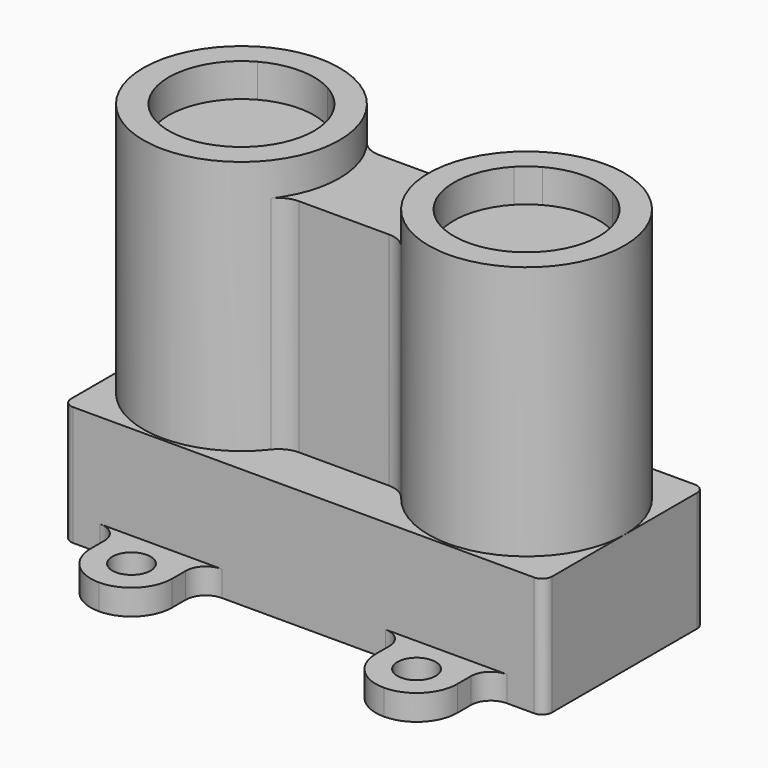
from build123d import *

# Parameters (mm, degrees)
F1_DEPTH    = 2.54
F2_DEPTH    = 11.938
F3_DEPTH    = 34
F4_DEPTH    = 37.338
F5_R        = 1
F6_R        = 2
F7_T1_DEPTH = 25.4067065919


# Not quite as in the source:
# - a fillet or chamfer that OpenCascade refuses, or shapes differently, is made with other operations: its cross-section is extruded or revolved along the edge and cut away or added


with BuildPart() as f1:
    # F0 (on Top) → F1 (new body)
    with BuildSketch(Plane.XY):
        with BuildLine():
            Line((16.129, 13.716), (18.288, 13.716))
            ThreePointArc((18.288, 13.716), (17.0976819587, 16.5896819587), (14.224, 17.78))
            ThreePointArc((14.224, 17.78), (11.3503180413, 16.5896819587), (10.16, 13.716))
            Line((10.16, 13.716), (12.319, 13.716))
            ThreePointArc((12.319, 13.716), (14.224, 15.621), (16.129, 13.716))
        make_face()
        with BuildLine():
            ThreePointArc((-10.16, 13.716), (-11.3503180413, 16.5896819587), (-14.224, 17.78))
            ThreePointArc((-14.224, 17.78), (-17.0976819587, 16.5896819587), (-18.288, 13.716))
            Line((-18.288, 13.716), (-16.129, 13.716))
            ThreePointArc((-16.129, 13.716), (-14.224, 15.621), (-12.319, 13.716))
            Line((-12.319, 13.716), (-10.16, 13.716))
        make_face()
        with BuildLine():
            ThreePointArc((-18.288, -13.716), (-17.0976819587, -16.5896819587), (-14.224, -17.78))
            ThreePointArc((-14.224, -17.78), (-11.3503180413, -16.5896819587), (-10.16, -13.716))
            Line((-10.16, -13.716), (-12.319, -13.716))
            ThreePointArc((-12.319, -13.716), (-14.224, -15.621), (-16.129, -13.716))
            Line((-16.129, -13.716), (-18.288, -13.716))
        make_face()
        with BuildLine():
            ThreePointArc((14.224, -17.78), (17.0976819587, -16.5896819587), (18.288, -13.716))
            Line((18.288, -13.716), (16.129, -13.716))
            ThreePointArc((16.129, -13.716), (14.224, -15.621), (12.319, -13.716))
            Line((12.319, -13.716), (10.16, -13.716))
            ThreePointArc((10.16, -13.716), (11.3503180413, -16.5896819587), (14.224, -17.78))
        make_face()
        with BuildLine():
            ThreePointArc((18.288, -13.716), (17.651692093, -11.5326486963), (15.9420241558, -10.033))
            Line((15.9420241558, -10.033), (12.5059758442, -10.033))
            ThreePointArc((12.5059758442, -10.033), (10.796307907, -11.5326486963), (10.16, -13.716))
            Line((10.16, -13.716), (12.319, -13.716))
            ThreePointArc((12.319, -13.716), (14.224, -11.811), (16.129, -13.716))
            Line((16.129, -13.716), (18.288, -13.716))
        make_face()
        with BuildLine():
            Line((18.288, -13.716), (18.288, -10.033))
            Line((18.288, -10.033), (15.9420241558, -10.033))
            ThreePointArc((15.9420241558, -10.033), (17.651692093, -11.5326486963), (18.288, -13.716))
        make_face()
        with BuildLine():
            ThreePointArc((10.16, -13.716), (10.796307907, -11.5326486963), (12.5059758442, -10.033))
            Line((12.5059758442, -10.033), (10.16, -10.033))
            Line((10.16, -10.033), (10.16, -13.716))
        make_face()
        with BuildLine():
            ThreePointArc((-15.9420241558, -10.033), (-17.651692093, -11.5326486963), (-18.288, -13.716))
            Line((-18.288, -13.716), (-16.129, -13.716))
            ThreePointArc((-16.129, -13.716), (-14.224, -11.811), (-12.319, -13.716))
            Line((-12.319, -13.716), (-10.16, -13.716))
            ThreePointArc((-10.16, -13.716), (-10.796307907, -11.5326486963), (-12.5059758442, -10.033))
            Line((-12.5059758442, -10.033), (-15.9420241558, -10.033))
        make_face()
        with BuildLine():
            Line((-18.288, -10.033), (-18.288, -13.716))
            ThreePointArc((-18.288, -13.716), (-17.651692093, -11.5326486963), (-15.9420241558, -10.033))
            Line((-15.9420241558, -10.033), (-18.288, -10.033))
        make_face()
        with BuildLine():
            ThreePointArc((-12.5059758442, -10.033), (-10.796307907, -11.5326486963), (-10.16, -13.716))
            Line((-10.16, -13.716), (-10.16, -10.033))
            Line((-10.16, -10.033), (-12.5059758442, -10.033))
        make_face()
        with BuildLine():
            Line((12.5059758442, 10.033), (15.9420241558, 10.033))
            ThreePointArc((15.9420241558, 10.033), (17.651692093, 11.5326486963), (18.288, 13.716))
            Line((18.288, 13.716), (16.129, 13.716))
            ThreePointArc((16.129, 13.716), (14.224, 11.811), (12.319, 13.716))
            Line((12.319, 13.716), (10.16, 13.716))
            ThreePointArc((10.16, 13.716), (10.796307907, 11.5326486963), (12.5059758442, 10.033))
        make_face()
        with BuildLine():
            ThreePointArc((-12.5059758442, 10.033), (-10.796307907, 11.5326486963), (-10.16, 13.716))
            Line((-10.16, 13.716), (-12.319, 13.716))
            ThreePointArc((-12.319, 13.716), (-14.224, 11.811), (-16.129, 13.716))
            Line((-16.129, 13.716), (-18.288, 13.716))
            ThreePointArc((-18.288, 13.716), (-17.651692093, 11.5326486963), (-15.9420241558, 10.033))
            Line((-15.9420241558, 10.033), (-12.5059758442, 10.033))
        make_face()
        with BuildLine():
            Line((-8.974, 5), (-5.8199033204, 5))
            ThreePointArc((-5.8199033204, 5), (-7.6929044902, 7.2782987326), (-10.16, 8.8945345578))
            Line((-10.16, 8.8945345578), (-10.16, 6.35))
            Line((-10.16, 6.35), (-10.7254288631, 6.35))
            ThreePointArc((-10.7254288631, 6.35), (-9.7979408912, 5.7421686466), (-8.974, 5))
        make_face()
        with BuildLine():
            Line((-17.7225711369, -6.35), (-10.7254288631, -6.35))
            ThreePointArc((-10.7254288631, -6.35), (-9.7979408912, -5.7421686466), (-8.974, -5))
            Line((-8.974, -5), (-9.5235463232, -5))
            Line((-9.5235463232, -5), (-9.5235463232, 5))
            Line((-9.5235463232, 5), (-8.974, 5))
            ThreePointArc((-8.974, 5), (-9.7979408912, 5.7421686466), (-10.7254288631, 6.35))
            Line((-10.7254288631, 6.35), (-17.7225711369, 6.35))
            ThreePointArc((-17.7225711369, 6.35), (-21.474, 0), (-17.7225711369, -6.35))
        make_face()
        with BuildLine():
            ThreePointArc((-18.288, 8.8945345578), (-22.4511105803, 5.2861604686), (-24.003, 0))
            ThreePointArc((-24.003, 0), (-22.4511105803, -5.2861604686), (-18.288, -8.8945345578))
            Line((-18.288, -8.8945345578), (-18.288, -6.35))
            Line((-18.288, -6.35), (-17.7225711369, -6.35))
            ThreePointArc((-17.7225711369, -6.35), (-21.474, 0), (-17.7225711369, 6.35))
            Line((-17.7225711369, 6.35), (-18.288, 6.35))
            Line((-18.288, 6.35), (-18.288, 8.8945345578))
        make_face()
        with BuildLine():
            ThreePointArc((-15.074346301, 9.7419583333), (-16.7174377184, 9.4557712189), (-18.288, 8.8945345578))
            Line((-18.288, 8.8945345578), (-18.288, 6.35))
            Line((-18.288, 6.35), (-17.7225711369, 6.35))
            ThreePointArc((-17.7225711369, 6.35), (-14.224, 7.25), (-10.7254288631, 6.35))
            Line((-10.7254288631, 6.35), (-10.16, 6.35))
            Line((-10.16, 6.35), (-10.16, 8.8945345578))
            ThreePointArc((-10.16, 8.8945345578), (-11.7305622816, 9.4557712189), (-13.373653699, 9.7419583333))
            ThreePointArc((-13.373653699, 9.7419583333), (-14.224, 9.652), (-15.074346301, 9.7419583333))
        make_face()
        with BuildLine():
            ThreePointArc((-13.373653699, -9.7419583333), (-11.7305622816, -9.4557712189), (-10.16, -8.8945345578))
            Line((-10.16, -8.8945345578), (-10.16, -6.35))
            Line((-10.16, -6.35), (-10.7254288631, -6.35))
            ThreePointArc((-10.7254288631, -6.35), (-14.224, -7.25), (-17.7225711369, -6.35))
            Line((-17.7225711369, -6.35), (-18.288, -6.35))
            Line((-18.288, -6.35), (-18.288, -8.8945345578))
            ThreePointArc((-18.288, -8.8945345578), (-16.7174377184, -9.4557712189), (-15.074346301, -9.7419583333))
            ThreePointArc((-15.074346301, -9.7419583333), (-14.224, -9.652), (-13.373653699, -9.7419583333))
        make_face()
        with BuildLine():
            ThreePointArc((15.074346301, -9.7419583333), (16.7174377184, -9.4557712189), (18.288, -8.8945345578))
            Line((18.288, -8.8945345578), (18.288, -6.35))
            Line((18.288, -6.35), (17.7225711369, -6.35))
            ThreePointArc((17.7225711369, -6.35), (14.224, -7.25), (10.7254288631, -6.35))
            Line((10.7254288631, -6.35), (10.16, -6.35))
            Line((10.16, -6.35), (10.16, -8.8945345578))
            ThreePointArc((10.16, -8.8945345578), (11.7305622816, -9.4557712189), (13.373653699, -9.7419583333))
            ThreePointArc((13.373653699, -9.7419583333), (14.224, -9.652), (15.074346301, -9.7419583333))
        make_face()
        with BuildLine():
            Line((18.288, 6.35), (18.288, 8.8945345578))
            ThreePointArc((18.288, 8.8945345578), (16.7174377184, 9.4557712189), (15.074346301, 9.7419583333))
            ThreePointArc((15.074346301, 9.7419583333), (14.224, 9.652), (13.373653699, 9.7419583333))
            ThreePointArc((13.373653699, 9.7419583333), (11.7305622816, 9.4557712189), (10.16, 8.8945345578))
            Line((10.16, 8.8945345578), (10.16, 6.35))
            Line((10.16, 6.35), (10.7254288631, 6.35))
            ThreePointArc((10.7254288631, 6.35), (14.224, 7.25), (17.7225711369, 6.35))
            Line((17.7225711369, 6.35), (18.288, 6.35))
        make_face()
        with BuildLine():
            Line((10.16, 10.033), (12.5059758442, 10.033))
            ThreePointArc((12.5059758442, 10.033), (10.796307907, 11.5326486963), (10.16, 13.716))
            Line((10.16, 13.716), (10.16, 10.033))
        make_face()
        with BuildLine():
            Line((15.9420241558, 10.033), (18.288, 10.033))
            Line((18.288, 10.033), (18.288, 13.716))
            ThreePointArc((18.288, 13.716), (17.651692093, 11.5326486963), (15.9420241558, 10.033))
        make_face()
        with BuildLine():
            ThreePointArc((13.373653699, 9.7419583333), (14.224, 9.779), (15.074346301, 9.7419583333))
            ThreePointArc((15.074346301, 9.7419583333), (15.5164039669, 9.8629767732), (15.9420241558, 10.033))
            Line((15.9420241558, 10.033), (12.5059758442, 10.033))
            ThreePointArc((12.5059758442, 10.033), (12.9315960331, 9.8629767732), (13.373653699, 9.7419583333))
        make_face()
        with BuildLine():
            Line((12.5059758442, -10.033), (15.9420241558, -10.033))
            ThreePointArc((15.9420241558, -10.033), (15.5164039669, -9.8629767732), (15.074346301, -9.7419583333))
            ThreePointArc((15.074346301, -9.7419583333), (14.224, -9.779), (13.373653699, -9.7419583333))
            ThreePointArc((13.373653699, -9.7419583333), (12.9315960331, -9.8629767732), (12.5059758442, -10.033))
        make_face()
        with BuildLine():
            ThreePointArc((-15.074346301, -9.7419583333), (-15.5164039669, -9.8629767732), (-15.9420241558, -10.033))
            Line((-15.9420241558, -10.033), (-12.5059758442, -10.033))
            ThreePointArc((-12.5059758442, -10.033), (-12.9315960331, -9.8629767732), (-13.373653699, -9.7419583333))
            ThreePointArc((-13.373653699, -9.7419583333), (-14.224, -9.779), (-15.074346301, -9.7419583333))
        make_face()
        with BuildLine():
            ThreePointArc((-13.373653699, 9.7419583333), (-12.9315960331, 9.8629767732), (-12.5059758442, 10.033))
            Line((-12.5059758442, 10.033), (-15.9420241558, 10.033))
            ThreePointArc((-15.9420241558, 10.033), (-15.5164039669, 9.8629767732), (-15.074346301, 9.7419583333))
            ThreePointArc((-15.074346301, 9.7419583333), (-14.224, 9.779), (-13.373653699, 9.7419583333))
        make_face()
        with BuildLine():
            ThreePointArc((-15.9420241558, 10.033), (-17.651692093, 11.5326486963), (-18.288, 13.716))
            Line((-18.288, 13.716), (-18.288, 10.033))
            Line((-18.288, 10.033), (-15.9420241558, 10.033))
        make_face()
        with BuildLine():
            Line((-10.16, 10.033), (-10.16, 13.716))
            ThreePointArc((-10.16, 13.716), (-10.796307907, 11.5326486963), (-12.5059758442, 10.033))
            Line((-12.5059758442, 10.033), (-10.16, 10.033))
        make_face()
        with BuildLine():
            Line((-9.5235463232, -5), (-8.974, -5))
            ThreePointArc((-8.974, -5), (-7.4925439911, -2.6925824036), (-6.974, 0))
            ThreePointArc((-6.974, 0), (-7.4925439911, 2.6925824036), (-8.974, 5))
            Line((-8.974, 5), (-9.5235463232, 5))
            Line((-9.5235463232, 5), (-9.5235463232, -5))
        make_face()
        with BuildLine():
            ThreePointArc((5.8199033204, 5), (7.6929044902, 7.2782987326), (10.16, 8.8945345578))
            Line((10.16, 8.8945345578), (10.16, 10.033))
            Line((10.16, 10.033), (-10.16, 10.033))
            Line((-10.16, 10.033), (-10.16, 8.8945345578))
            ThreePointArc((-10.16, 8.8945345578), (-7.6929044902, 7.2782987326), (-5.8199033204, 5))
            Line((-5.8199033204, 5), (5.8199033204, 5))
        make_face()
        with BuildLine():
            ThreePointArc((8.974, 5), (6.974, 0), (8.974, -5))
            Line((8.974, -5), (9.5235463232, -5))
            Line((9.5235463232, -5), (9.5235463232, 5))
            Line((9.5235463232, 5), (8.974, 5))
        make_face()
        with BuildLine():
            Line((-5.8199033204, -5), (5.8199033204, -5))
            ThreePointArc((5.8199033204, -5), (4.445, 0), (5.8199033204, 5))
            Line((5.8199033204, 5), (-5.8199033204, 5))
            ThreePointArc((-5.8199033204, 5), (-4.7949888528, 2.5927957469), (-4.445, 0))
            ThreePointArc((-4.445, 0), (-4.7949888528, -2.5927957469), (-5.8199033204, -5))
        make_face()
        with BuildLine():
            Line((-10.16, -10.033), (10.16, -10.033))
            Line((10.16, -10.033), (10.16, -8.8945345578))
            ThreePointArc((10.16, -8.8945345578), (7.6929044902, -7.2782987326), (5.8199033204, -5))
            Line((5.8199033204, -5), (-5.8199033204, -5))
            ThreePointArc((-5.8199033204, -5), (-7.6929044902, -7.2782987326), (-10.16, -8.8945345578))
            Line((-10.16, -8.8945345578), (-10.16, -10.033))
        make_face()
        with BuildLine():
            ThreePointArc((18.288, -8.8945345578), (22.4511105803, -5.2861604686), (24.003, 0))
            ThreePointArc((24.003, 0), (22.4511105803, 5.2861604686), (18.288, 8.8945345578))
            Line((18.288, 8.8945345578), (18.288, 6.35))
            Line((18.288, 6.35), (17.7225711369, 6.35))
            ThreePointArc((17.7225711369, 6.35), (20.4660806124, 3.6876726575), (21.474, 0))
            ThreePointArc((21.474, 0), (20.4660806124, -3.6876726575), (17.7225711369, -6.35))
            Line((17.7225711369, -6.35), (18.288, -6.35))
            Line((18.288, -6.35), (18.288, -8.8945345578))
        make_face()
        with BuildLine():
            Line((10.7254288631, -6.35), (17.7225711369, -6.35))
            ThreePointArc((17.7225711369, -6.35), (20.4660806124, -3.6876726575), (21.474, 0))
            ThreePointArc((21.474, 0), (20.4660806124, 3.6876726575), (17.7225711369, 6.35))
            Line((17.7225711369, 6.35), (10.7254288631, 6.35))
            ThreePointArc((10.7254288631, 6.35), (9.7979408912, 5.7421686466), (8.974, 5))
            Line((8.974, 5), (9.5235463232, 5))
            Line((9.5235463232, 5), (9.5235463232, -5))
            Line((9.5235463232, -5), (8.974, -5))
            ThreePointArc((8.974, -5), (9.7979408912, -5.7421686466), (10.7254288631, -6.35))
        make_face()
        with BuildLine():
            ThreePointArc((8.974, 5), (9.7979408912, 5.7421686466), (10.7254288631, 6.35))
            Line((10.7254288631, 6.35), (10.16, 6.35))
            Line((10.16, 6.35), (10.16, 8.8945345578))
            ThreePointArc((10.16, 8.8945345578), (7.6929044902, 7.2782987326), (5.8199033204, 5))
            Line((5.8199033204, 5), (8.974, 5))
        make_face()
        with BuildLine():
            ThreePointArc((-15.074346301, 9.7419583333), (-15.5164039669, 9.8629767732), (-15.9420241558, 10.033))
            Line((-15.9420241558, 10.033), (-18.288, 10.033))
            Line((-18.288, 10.033), (-18.288, 8.8945345578))
            ThreePointArc((-18.288, 8.8945345578), (-16.7174377184, 9.4557712189), (-15.074346301, 9.7419583333))
        make_face()
        with BuildLine():
            ThreePointArc((-15.074346301, 9.7419583333), (-14.224, 9.652), (-13.373653699, 9.7419583333))
            ThreePointArc((-13.373653699, 9.7419583333), (-14.224, 9.779), (-15.074346301, 9.7419583333))
        make_face()
        with BuildLine():
            Line((-10.16, 8.8945345578), (-10.16, 10.033))
            Line((-10.16, 10.033), (-12.5059758442, 10.033))
            ThreePointArc((-12.5059758442, 10.033), (-12.9315960331, 9.8629767732), (-13.373653699, 9.7419583333))
            ThreePointArc((-13.373653699, 9.7419583333), (-11.7305622816, 9.4557712189), (-10.16, 8.8945345578))
        make_face()
        with BuildLine():
            Line((-18.288, -10.033), (-15.9420241558, -10.033))
            ThreePointArc((-15.9420241558, -10.033), (-15.5164039669, -9.8629767732), (-15.074346301, -9.7419583333))
            ThreePointArc((-15.074346301, -9.7419583333), (-16.7174377184, -9.4557712189), (-18.288, -8.8945345578))
            Line((-18.288, -8.8945345578), (-18.288, -10.033))
        make_face()
        with BuildLine():
            ThreePointArc((-13.373653699, -9.7419583333), (-14.224, -9.652), (-15.074346301, -9.7419583333))
            ThreePointArc((-15.074346301, -9.7419583333), (-14.224, -9.779), (-13.373653699, -9.7419583333))
        make_face()
        with BuildLine():
            Line((-12.5059758442, -10.033), (-10.16, -10.033))
            Line((-10.16, -10.033), (-10.16, -8.8945345578))
            ThreePointArc((-10.16, -8.8945345578), (-11.7305622816, -9.4557712189), (-13.373653699, -9.7419583333))
            ThreePointArc((-13.373653699, -9.7419583333), (-12.9315960331, -9.8629767732), (-12.5059758442, -10.033))
        make_face()
        with BuildLine():
            Line((15.9420241558, -10.033), (18.288, -10.033))
            Line((18.288, -10.033), (18.288, -8.8945345578))
            ThreePointArc((18.288, -8.8945345578), (16.7174377184, -9.4557712189), (15.074346301, -9.7419583333))
            ThreePointArc((15.074346301, -9.7419583333), (15.5164039669, -9.8629767732), (15.9420241558, -10.033))
        make_face()
        with BuildLine():
            Line((10.16, -10.033), (12.5059758442, -10.033))
            ThreePointArc((12.5059758442, -10.033), (12.9315960331, -9.8629767732), (13.373653699, -9.7419583333))
            ThreePointArc((13.373653699, -9.7419583333), (11.7305622816, -9.4557712189), (10.16, -8.8945345578))
            Line((10.16, -8.8945345578), (10.16, -10.033))
        make_face()
        with BuildLine():
            ThreePointArc((13.373653699, -9.7419583333), (14.224, -9.779), (15.074346301, -9.7419583333))
            ThreePointArc((15.074346301, -9.7419583333), (14.224, -9.652), (13.373653699, -9.7419583333))
        make_face()
        with BuildLine():
            ThreePointArc((13.373653699, 9.7419583333), (14.224, 9.652), (15.074346301, 9.7419583333))
            ThreePointArc((15.074346301, 9.7419583333), (14.224, 9.779), (13.373653699, 9.7419583333))
        make_face()
        with BuildLine():
            ThreePointArc((10.16, 8.8945345578), (11.7305622816, 9.4557712189), (13.373653699, 9.7419583333))
            ThreePointArc((13.373653699, 9.7419583333), (12.9315960331, 9.8629767732), (12.5059758442, 10.033))
            Line((12.5059758442, 10.033), (10.16, 10.033))
            Line((10.16, 10.033), (10.16, 8.8945345578))
        make_face()
        with BuildLine():
            ThreePointArc((15.074346301, 9.7419583333), (16.7174377184, 9.4557712189), (18.288, 8.8945345578))
            Line((18.288, 8.8945345578), (18.288, 10.033))
            Line((18.288, 10.033), (15.9420241558, 10.033))
            ThreePointArc((15.9420241558, 10.033), (15.5164039669, 9.8629767732), (15.074346301, 9.7419583333))
        make_face()
        with BuildLine():
            Line((18.288, -10.033), (24.003, -10.033))
            Line((24.003, -10.033), (24.003, 0))
            ThreePointArc((24.003, 0), (22.4511105803, -5.2861604686), (18.288, -8.8945345578))
            Line((18.288, -8.8945345578), (18.288, -10.033))
        make_face()
        with BuildLine():
            ThreePointArc((18.288, 8.8945345578), (22.4511105803, 5.2861604686), (24.003, 0))
            Line((24.003, 0), (24.003, 10.033))
            Line((24.003, 10.033), (18.288, 10.033))
            Line((18.288, 10.033), (18.288, 8.8945345578))
        make_face()
        with BuildLine():
            Line((-24.003, 0), (-24.003, -10.033))
            Line((-24.003, -10.033), (-18.288, -10.033))
            Line((-18.288, -10.033), (-18.288, -8.8945345578))
            ThreePointArc((-18.288, -8.8945345578), (-22.4511105803, -5.2861604686), (-24.003, 0))
        make_face()
        with BuildLine():
            Line((-24.003, 10.033), (-24.003, 0))
            ThreePointArc((-24.003, 0), (-22.4511105803, 5.2861604686), (-18.288, 8.8945345578))
            Line((-18.288, 8.8945345578), (-18.288, 10.033))
            Line((-18.288, 10.033), (-24.003, 10.033))
        make_face()
        with BuildLine():
            Line((-8.974, -5), (-5.8199033204, -5))
            ThreePointArc((-5.8199033204, -5), (-4.7949888528, -2.5927957469), (-4.445, 0))
            ThreePointArc((-4.445, 0), (-4.7949888528, 2.5927957469), (-5.8199033204, 5))
            Line((-5.8199033204, 5), (-8.974, 5))
            ThreePointArc((-8.974, 5), (-7.4925439911, 2.6925824036), (-6.974, 0))
            ThreePointArc((-6.974, 0), (-7.4925439911, -2.6925824036), (-8.974, -5))
        make_face()
        with BuildLine():
            ThreePointArc((-17.7225711369, -6.35), (-14.224, -7.25), (-10.7254288631, -6.35))
            Line((-10.7254288631, -6.35), (-17.7225711369, -6.35))
        make_face()
        with BuildLine():
            Line((-17.7225711369, 6.35), (-10.7254288631, 6.35))
            ThreePointArc((-10.7254288631, 6.35), (-14.224, 7.25), (-17.7225711369, 6.35))
        make_face()
        with BuildLine():
            Line((-10.16, -6.35), (-10.16, -8.8945345578))
            ThreePointArc((-10.16, -8.8945345578), (-7.6929044902, -7.2782987326), (-5.8199033204, -5))
            Line((-5.8199033204, -5), (-8.974, -5))
            ThreePointArc((-8.974, -5), (-9.7979408912, -5.7421686466), (-10.7254288631, -6.35))
            Line((-10.7254288631, -6.35), (-10.16, -6.35))
        make_face()
        with BuildLine():
            ThreePointArc((5.8199033204, 5), (4.445, 0), (5.8199033204, -5))
            Line((5.8199033204, -5), (8.974, -5))
            ThreePointArc((8.974, -5), (6.974, 0), (8.974, 5))
            Line((8.974, 5), (5.8199033204, 5))
        make_face()
        with BuildLine():
            ThreePointArc((5.8199033204, -5), (7.6929044902, -7.2782987326), (10.16, -8.8945345578))
            Line((10.16, -8.8945345578), (10.16, -6.35))
            Line((10.16, -6.35), (10.7254288631, -6.35))
            ThreePointArc((10.7254288631, -6.35), (9.7979408912, -5.7421686466), (8.974, -5))
            Line((8.974, -5), (5.8199033204, -5))
        make_face()
        with BuildLine():
            ThreePointArc((10.7254288631, -6.35), (14.224, -7.25), (17.7225711369, -6.35))
            Line((17.7225711369, -6.35), (10.7254288631, -6.35))
        make_face()
        with BuildLine():
            Line((10.7254288631, 6.35), (17.7225711369, 6.35))
            ThreePointArc((17.7225711369, 6.35), (14.224, 7.25), (10.7254288631, 6.35))
        make_face()
    extrude(amount=F1_DEPTH)

    # F0 (on Top) → F2 (join)
    with BuildSketch(Plane.XY):
        with BuildLine():
            Line((-8.974, 5), (-5.8199033204, 5))
            ThreePointArc((-5.8199033204, 5), (-7.6929044902, 7.2782987326), (-10.16, 8.8945345578))
            Line((-10.16, 8.8945345578), (-10.16, 6.35))
            Line((-10.16, 6.35), (-10.7254288631, 6.35))
            ThreePointArc((-10.7254288631, 6.35), (-9.7979408912, 5.7421686466), (-8.974, 5))
        make_face()
        with BuildLine():
            Line((-17.7225711369, -6.35), (-10.7254288631, -6.35))
            ThreePointArc((-10.7254288631, -6.35), (-9.7979408912, -5.7421686466), (-8.974, -5))
            Line((-8.974, -5), (-9.5235463232, -5))
            Line((-9.5235463232, -5), (-9.5235463232, 5))
            Line((-9.5235463232, 5), (-8.974, 5))
            ThreePointArc((-8.974, 5), (-9.7979408912, 5.7421686466), (-10.7254288631, 6.35))
            Line((-10.7254288631, 6.35), (-17.7225711369, 6.35))
            ThreePointArc((-17.7225711369, 6.35), (-21.474, 0), (-17.7225711369, -6.35))
        make_face()
        with BuildLine():
            ThreePointArc((-18.288, 8.8945345578), (-22.4511105803, 5.2861604686), (-24.003, 0))
            ThreePointArc((-24.003, 0), (-22.4511105803, -5.2861604686), (-18.288, -8.8945345578))
            Line((-18.288, -8.8945345578), (-18.288, -6.35))
            Line((-18.288, -6.35), (-17.7225711369, -6.35))
            ThreePointArc((-17.7225711369, -6.35), (-21.474, 0), (-17.7225711369, 6.35))
            Line((-17.7225711369, 6.35), (-18.288, 6.35))
            Line((-18.288, 6.35), (-18.288, 8.8945345578))
        make_face()
        with BuildLine():
            ThreePointArc((-13.373653699, -9.7419583333), (-11.7305622816, -9.4557712189), (-10.16, -8.8945345578))
            Line((-10.16, -8.8945345578), (-10.16, -6.35))
            Line((-10.16, -6.35), (-10.7254288631, -6.35))
            ThreePointArc((-10.7254288631, -6.35), (-14.224, -7.25), (-17.7225711369, -6.35))
            Line((-17.7225711369, -6.35), (-18.288, -6.35))
            Line((-18.288, -6.35), (-18.288, -8.8945345578))
            ThreePointArc((-18.288, -8.8945345578), (-16.7174377184, -9.4557712189), (-15.074346301, -9.7419583333))
            ThreePointArc((-15.074346301, -9.7419583333), (-14.224, -9.652), (-13.373653699, -9.7419583333))
        make_face()
        with BuildLine():
            ThreePointArc((15.074346301, -9.7419583333), (16.7174377184, -9.4557712189), (18.288, -8.8945345578))
            Line((18.288, -8.8945345578), (18.288, -6.35))
            Line((18.288, -6.35), (17.7225711369, -6.35))
            ThreePointArc((17.7225711369, -6.35), (14.224, -7.25), (10.7254288631, -6.35))
            Line((10.7254288631, -6.35), (10.16, -6.35))
            Line((10.16, -6.35), (10.16, -8.8945345578))
            ThreePointArc((10.16, -8.8945345578), (11.7305622816, -9.4557712189), (13.373653699, -9.7419583333))
            ThreePointArc((13.373653699, -9.7419583333), (14.224, -9.652), (15.074346301, -9.7419583333))
        make_face()
        with BuildLine():
            Line((18.288, 6.35), (18.288, 8.8945345578))
            ThreePointArc((18.288, 8.8945345578), (16.7174377184, 9.4557712189), (15.074346301, 9.7419583333))
            ThreePointArc((15.074346301, 9.7419583333), (14.224, 9.652), (13.373653699, 9.7419583333))
            ThreePointArc((13.373653699, 9.7419583333), (11.7305622816, 9.4557712189), (10.16, 8.8945345578))
            Line((10.16, 8.8945345578), (10.16, 6.35))
            Line((10.16, 6.35), (10.7254288631, 6.35))
            ThreePointArc((10.7254288631, 6.35), (14.224, 7.25), (17.7225711369, 6.35))
            Line((17.7225711369, 6.35), (18.288, 6.35))
        make_face()
        with BuildLine():
            Line((12.5059758442, -10.033), (15.9420241558, -10.033))
            ThreePointArc((15.9420241558, -10.033), (15.5164039669, -9.8629767732), (15.074346301, -9.7419583333))
            ThreePointArc((15.074346301, -9.7419583333), (14.224, -9.779), (13.373653699, -9.7419583333))
            ThreePointArc((13.373653699, -9.7419583333), (12.9315960331, -9.8629767732), (12.5059758442, -10.033))
        make_face()
        with BuildLine():
            ThreePointArc((13.373653699, 9.7419583333), (14.224, 9.779), (15.074346301, 9.7419583333))
            ThreePointArc((15.074346301, 9.7419583333), (15.5164039669, 9.8629767732), (15.9420241558, 10.033))
            Line((15.9420241558, 10.033), (12.5059758442, 10.033))
            ThreePointArc((12.5059758442, 10.033), (12.9315960331, 9.8629767732), (13.373653699, 9.7419583333))
        make_face()
        with BuildLine():
            ThreePointArc((-15.074346301, -9.7419583333), (-15.5164039669, -9.8629767732), (-15.9420241558, -10.033))
            Line((-15.9420241558, -10.033), (-12.5059758442, -10.033))
            ThreePointArc((-12.5059758442, -10.033), (-12.9315960331, -9.8629767732), (-13.373653699, -9.7419583333))
            ThreePointArc((-13.373653699, -9.7419583333), (-14.224, -9.779), (-15.074346301, -9.7419583333))
        make_face()
        with BuildLine():
            ThreePointArc((-13.373653699, 9.7419583333), (-12.9315960331, 9.8629767732), (-12.5059758442, 10.033))
            Line((-12.5059758442, 10.033), (-15.9420241558, 10.033))
            ThreePointArc((-15.9420241558, 10.033), (-15.5164039669, 9.8629767732), (-15.074346301, 9.7419583333))
            ThreePointArc((-15.074346301, 9.7419583333), (-14.224, 9.779), (-13.373653699, 9.7419583333))
        make_face()
        with BuildLine():
            Line((-24.003, 10.033), (-24.003, 0))
            ThreePointArc((-24.003, 0), (-22.4511105803, 5.2861604686), (-18.288, 8.8945345578))
            Line((-18.288, 8.8945345578), (-18.288, 10.033))
            Line((-18.288, 10.033), (-24.003, 10.033))
        make_face()
        with BuildLine():
            Line((-24.003, 0), (-24.003, -10.033))
            Line((-24.003, -10.033), (-18.288, -10.033))
            Line((-18.288, -10.033), (-18.288, -8.8945345578))
            ThreePointArc((-18.288, -8.8945345578), (-22.4511105803, -5.2861604686), (-24.003, 0))
        make_face()
        with BuildLine():
            Line((-10.16, -10.033), (10.16, -10.033))
            Line((10.16, -10.033), (10.16, -8.8945345578))
            ThreePointArc((10.16, -8.8945345578), (7.6929044902, -7.2782987326), (5.8199033204, -5))
            Line((5.8199033204, -5), (-5.8199033204, -5))
            ThreePointArc((-5.8199033204, -5), (-7.6929044902, -7.2782987326), (-10.16, -8.8945345578))
            Line((-10.16, -8.8945345578), (-10.16, -10.033))
        make_face()
        with BuildLine():
            Line((-9.5235463232, -5), (-8.974, -5))
            ThreePointArc((-8.974, -5), (-7.4925439911, -2.6925824036), (-6.974, 0))
            ThreePointArc((-6.974, 0), (-7.4925439911, 2.6925824036), (-8.974, 5))
            Line((-8.974, 5), (-9.5235463232, 5))
            Line((-9.5235463232, 5), (-9.5235463232, -5))
        make_face()
        with BuildLine():
            Line((-5.8199033204, -5), (5.8199033204, -5))
            ThreePointArc((5.8199033204, -5), (4.445, 0), (5.8199033204, 5))
            Line((5.8199033204, 5), (-5.8199033204, 5))
            ThreePointArc((-5.8199033204, 5), (-4.7949888528, 2.5927957469), (-4.445, 0))
            ThreePointArc((-4.445, 0), (-4.7949888528, -2.5927957469), (-5.8199033204, -5))
        make_face()
        with BuildLine():
            ThreePointArc((8.974, 5), (6.974, 0), (8.974, -5))
            Line((8.974, -5), (9.5235463232, -5))
            Line((9.5235463232, -5), (9.5235463232, 5))
            Line((9.5235463232, 5), (8.974, 5))
        make_face()
        with BuildLine():
            ThreePointArc((18.288, -8.8945345578), (22.4511105803, -5.2861604686), (24.003, 0))
            ThreePointArc((24.003, 0), (22.4511105803, 5.2861604686), (18.288, 8.8945345578))
            Line((18.288, 8.8945345578), (18.288, 6.35))
            Line((18.288, 6.35), (17.7225711369, 6.35))
            ThreePointArc((17.7225711369, 6.35), (20.4660806124, 3.6876726575), (21.474, 0))
            ThreePointArc((21.474, 0), (20.4660806124, -3.6876726575), (17.7225711369, -6.35))
            Line((17.7225711369, -6.35), (18.288, -6.35))
            Line((18.288, -6.35), (18.288, -8.8945345578))
        make_face()
        with BuildLine():
            Line((10.7254288631, -6.35), (17.7225711369, -6.35))
            ThreePointArc((17.7225711369, -6.35), (20.4660806124, -3.6876726575), (21.474, 0))
            ThreePointArc((21.474, 0), (20.4660806124, 3.6876726575), (17.7225711369, 6.35))
            Line((17.7225711369, 6.35), (10.7254288631, 6.35))
            ThreePointArc((10.7254288631, 6.35), (9.7979408912, 5.7421686466), (8.974, 5))
            Line((8.974, 5), (9.5235463232, 5))
            Line((9.5235463232, 5), (9.5235463232, -5))
            Line((9.5235463232, -5), (8.974, -5))
            ThreePointArc((8.974, -5), (9.7979408912, -5.7421686466), (10.7254288631, -6.35))
        make_face()
        with BuildLine():
            ThreePointArc((8.974, 5), (9.7979408912, 5.7421686466), (10.7254288631, 6.35))
            Line((10.7254288631, 6.35), (10.16, 6.35))
            Line((10.16, 6.35), (10.16, 8.8945345578))
            ThreePointArc((10.16, 8.8945345578), (7.6929044902, 7.2782987326), (5.8199033204, 5))
            Line((5.8199033204, 5), (8.974, 5))
        make_face()
        with BuildLine():
            ThreePointArc((18.288, 8.8945345578), (22.4511105803, 5.2861604686), (24.003, 0))
            Line((24.003, 0), (24.003, 10.033))
            Line((24.003, 10.033), (18.288, 10.033))
            Line((18.288, 10.033), (18.288, 8.8945345578))
        make_face()
        with BuildLine():
            Line((18.288, -10.033), (24.003, -10.033))
            Line((24.003, -10.033), (24.003, 0))
            ThreePointArc((24.003, 0), (22.4511105803, -5.2861604686), (18.288, -8.8945345578))
            Line((18.288, -8.8945345578), (18.288, -10.033))
        make_face()
        with BuildLine():
            ThreePointArc((5.8199033204, 5), (7.6929044902, 7.2782987326), (10.16, 8.8945345578))
            Line((10.16, 8.8945345578), (10.16, 10.033))
            Line((10.16, 10.033), (-10.16, 10.033))
            Line((-10.16, 10.033), (-10.16, 8.8945345578))
            ThreePointArc((-10.16, 8.8945345578), (-7.6929044902, 7.2782987326), (-5.8199033204, 5))
            Line((-5.8199033204, 5), (5.8199033204, 5))
        make_face()
        with BuildLine():
            Line((-12.5059758442, -10.033), (-10.16, -10.033))
            Line((-10.16, -10.033), (-10.16, -8.8945345578))
            ThreePointArc((-10.16, -8.8945345578), (-11.7305622816, -9.4557712189), (-13.373653699, -9.7419583333))
            ThreePointArc((-13.373653699, -9.7419583333), (-12.9315960331, -9.8629767732), (-12.5059758442, -10.033))
        make_face()
        with BuildLine():
            Line((-18.288, -10.033), (-15.9420241558, -10.033))
            ThreePointArc((-15.9420241558, -10.033), (-15.5164039669, -9.8629767732), (-15.074346301, -9.7419583333))
            ThreePointArc((-15.074346301, -9.7419583333), (-16.7174377184, -9.4557712189), (-18.288, -8.8945345578))
            Line((-18.288, -8.8945345578), (-18.288, -10.033))
        make_face()
        with BuildLine():
            ThreePointArc((-13.373653699, -9.7419583333), (-14.224, -9.652), (-15.074346301, -9.7419583333))
            ThreePointArc((-15.074346301, -9.7419583333), (-14.224, -9.779), (-13.373653699, -9.7419583333))
        make_face()
        with BuildLine():
            Line((-10.16, 8.8945345578), (-10.16, 10.033))
            Line((-10.16, 10.033), (-12.5059758442, 10.033))
            ThreePointArc((-12.5059758442, 10.033), (-12.9315960331, 9.8629767732), (-13.373653699, 9.7419583333))
            ThreePointArc((-13.373653699, 9.7419583333), (-11.7305622816, 9.4557712189), (-10.16, 8.8945345578))
        make_face()
        with BuildLine():
            ThreePointArc((-15.074346301, 9.7419583333), (-15.5164039669, 9.8629767732), (-15.9420241558, 10.033))
            Line((-15.9420241558, 10.033), (-18.288, 10.033))
            Line((-18.288, 10.033), (-18.288, 8.8945345578))
            ThreePointArc((-18.288, 8.8945345578), (-16.7174377184, 9.4557712189), (-15.074346301, 9.7419583333))
        make_face()
        with BuildLine():
            ThreePointArc((-15.074346301, 9.7419583333), (-14.224, 9.652), (-13.373653699, 9.7419583333))
            ThreePointArc((-13.373653699, 9.7419583333), (-14.224, 9.779), (-15.074346301, 9.7419583333))
        make_face()
        with BuildLine():
            ThreePointArc((-15.074346301, 9.7419583333), (-16.7174377184, 9.4557712189), (-18.288, 8.8945345578))
            Line((-18.288, 8.8945345578), (-18.288, 6.35))
            Line((-18.288, 6.35), (-17.7225711369, 6.35))
            ThreePointArc((-17.7225711369, 6.35), (-14.224, 7.25), (-10.7254288631, 6.35))
            Line((-10.7254288631, 6.35), (-10.16, 6.35))
            Line((-10.16, 6.35), (-10.16, 8.8945345578))
            ThreePointArc((-10.16, 8.8945345578), (-11.7305622816, 9.4557712189), (-13.373653699, 9.7419583333))
            ThreePointArc((-13.373653699, 9.7419583333), (-14.224, 9.652), (-15.074346301, 9.7419583333))
        make_face()
        with BuildLine():
            Line((15.9420241558, -10.033), (18.288, -10.033))
            Line((18.288, -10.033), (18.288, -8.8945345578))
            ThreePointArc((18.288, -8.8945345578), (16.7174377184, -9.4557712189), (15.074346301, -9.7419583333))
            ThreePointArc((15.074346301, -9.7419583333), (15.5164039669, -9.8629767732), (15.9420241558, -10.033))
        make_face()
        with BuildLine():
            Line((10.16, -10.033), (12.5059758442, -10.033))
            ThreePointArc((12.5059758442, -10.033), (12.9315960331, -9.8629767732), (13.373653699, -9.7419583333))
            ThreePointArc((13.373653699, -9.7419583333), (11.7305622816, -9.4557712189), (10.16, -8.8945345578))
            Line((10.16, -8.8945345578), (10.16, -10.033))
        make_face()
        with BuildLine():
            ThreePointArc((13.373653699, -9.7419583333), (14.224, -9.779), (15.074346301, -9.7419583333))
            ThreePointArc((15.074346301, -9.7419583333), (14.224, -9.652), (13.373653699, -9.7419583333))
        make_face()
        with BuildLine():
            ThreePointArc((15.074346301, 9.7419583333), (16.7174377184, 9.4557712189), (18.288, 8.8945345578))
            Line((18.288, 8.8945345578), (18.288, 10.033))
            Line((18.288, 10.033), (15.9420241558, 10.033))
            ThreePointArc((15.9420241558, 10.033), (15.5164039669, 9.8629767732), (15.074346301, 9.7419583333))
        make_face()
        with BuildLine():
            ThreePointArc((10.16, 8.8945345578), (11.7305622816, 9.4557712189), (13.373653699, 9.7419583333))
            ThreePointArc((13.373653699, 9.7419583333), (12.9315960331, 9.8629767732), (12.5059758442, 10.033))
            Line((12.5059758442, 10.033), (10.16, 10.033))
            Line((10.16, 10.033), (10.16, 8.8945345578))
        make_face()
        with BuildLine():
            ThreePointArc((13.373653699, 9.7419583333), (14.224, 9.652), (15.074346301, 9.7419583333))
            ThreePointArc((15.074346301, 9.7419583333), (14.224, 9.779), (13.373653699, 9.7419583333))
        make_face()
        with BuildLine():
            Line((-17.7225711369, 6.35), (-10.7254288631, 6.35))
            ThreePointArc((-10.7254288631, 6.35), (-14.224, 7.25), (-17.7225711369, 6.35))
        make_face()
        with BuildLine():
            ThreePointArc((-17.7225711369, -6.35), (-14.224, -7.25), (-10.7254288631, -6.35))
            Line((-10.7254288631, -6.35), (-17.7225711369, -6.35))
        make_face()
        with BuildLine():
            Line((-8.974, -5), (-5.8199033204, -5))
            ThreePointArc((-5.8199033204, -5), (-4.7949888528, -2.5927957469), (-4.445, 0))
            ThreePointArc((-4.445, 0), (-4.7949888528, 2.5927957469), (-5.8199033204, 5))
            Line((-5.8199033204, 5), (-8.974, 5))
            ThreePointArc((-8.974, 5), (-7.4925439911, 2.6925824036), (-6.974, 0))
            ThreePointArc((-6.974, 0), (-7.4925439911, -2.6925824036), (-8.974, -5))
        make_face()
        with BuildLine():
            ThreePointArc((5.8199033204, 5), (4.445, 0), (5.8199033204, -5))
            Line((5.8199033204, -5), (8.974, -5))
            ThreePointArc((8.974, -5), (6.974, 0), (8.974, 5))
            Line((8.974, 5), (5.8199033204, 5))
        make_face()
        with BuildLine():
            Line((10.7254288631, 6.35), (17.7225711369, 6.35))
            ThreePointArc((17.7225711369, 6.35), (14.224, 7.25), (10.7254288631, 6.35))
        make_face()
        with BuildLine():
            ThreePointArc((10.7254288631, -6.35), (14.224, -7.25), (17.7225711369, -6.35))
            Line((17.7225711369, -6.35), (10.7254288631, -6.35))
        make_face()
        with BuildLine():
            ThreePointArc((5.8199033204, -5), (7.6929044902, -7.2782987326), (10.16, -8.8945345578))
            Line((10.16, -8.8945345578), (10.16, -6.35))
            Line((10.16, -6.35), (10.7254288631, -6.35))
            ThreePointArc((10.7254288631, -6.35), (9.7979408912, -5.7421686466), (8.974, -5))
            Line((8.974, -5), (5.8199033204, -5))
        make_face()
        with BuildLine():
            Line((-10.16, -6.35), (-10.16, -8.8945345578))
            ThreePointArc((-10.16, -8.8945345578), (-7.6929044902, -7.2782987326), (-5.8199033204, -5))
            Line((-5.8199033204, -5), (-8.974, -5))
            ThreePointArc((-8.974, -5), (-9.7979408912, -5.7421686466), (-10.7254288631, -6.35))
            Line((-10.7254288631, -6.35), (-10.16, -6.35))
        make_face()
    extrude(amount=F2_DEPTH)

    # F0 (on Top) → F3 (join)
    with BuildSketch(Plane.XY):
        with BuildLine():
            ThreePointArc((-18.288, 8.8945345578), (-22.4511105803, 5.2861604686), (-24.003, 0))
            ThreePointArc((-24.003, 0), (-22.4511105803, -5.2861604686), (-18.288, -8.8945345578))
            Line((-18.288, -8.8945345578), (-18.288, -6.35))
            Line((-18.288, -6.35), (-17.7225711369, -6.35))
            ThreePointArc((-17.7225711369, -6.35), (-21.474, 0), (-17.7225711369, 6.35))
            Line((-17.7225711369, 6.35), (-18.288, 6.35))
            Line((-18.288, 6.35), (-18.288, 8.8945345578))
        make_face()
        with BuildLine():
            ThreePointArc((-15.074346301, 9.7419583333), (-16.7174377184, 9.4557712189), (-18.288, 8.8945345578))
            Line((-18.288, 8.8945345578), (-18.288, 6.35))
            Line((-18.288, 6.35), (-17.7225711369, 6.35))
            ThreePointArc((-17.7225711369, 6.35), (-14.224, 7.25), (-10.7254288631, 6.35))
            Line((-10.7254288631, 6.35), (-10.16, 6.35))
            Line((-10.16, 6.35), (-10.16, 8.8945345578))
            ThreePointArc((-10.16, 8.8945345578), (-11.7305622816, 9.4557712189), (-13.373653699, 9.7419583333))
            ThreePointArc((-13.373653699, 9.7419583333), (-14.224, 9.652), (-15.074346301, 9.7419583333))
        make_face()
        with BuildLine():
            Line((-8.974, 5), (-5.8199033204, 5))
            ThreePointArc((-5.8199033204, 5), (-7.6929044902, 7.2782987326), (-10.16, 8.8945345578))
            Line((-10.16, 8.8945345578), (-10.16, 6.35))
            Line((-10.16, 6.35), (-10.7254288631, 6.35))
            ThreePointArc((-10.7254288631, 6.35), (-9.7979408912, 5.7421686466), (-8.974, 5))
        make_face()
        with BuildLine():
            Line((-8.974, -5), (-5.8199033204, -5))
            ThreePointArc((-5.8199033204, -5), (-4.7949888528, -2.5927957469), (-4.445, 0))
            ThreePointArc((-4.445, 0), (-4.7949888528, 2.5927957469), (-5.8199033204, 5))
            Line((-5.8199033204, 5), (-8.974, 5))
            ThreePointArc((-8.974, 5), (-7.4925439911, 2.6925824036), (-6.974, 0))
            ThreePointArc((-6.974, 0), (-7.4925439911, -2.6925824036), (-8.974, -5))
        make_face()
        with BuildLine():
            Line((-5.8199033204, -5), (5.8199033204, -5))
            ThreePointArc((5.8199033204, -5), (4.445, 0), (5.8199033204, 5))
            Line((5.8199033204, 5), (-5.8199033204, 5))
            ThreePointArc((-5.8199033204, 5), (-4.7949888528, 2.5927957469), (-4.445, 0))
            ThreePointArc((-4.445, 0), (-4.7949888528, -2.5927957469), (-5.8199033204, -5))
        make_face()
        with BuildLine():
            Line((-10.16, -6.35), (-10.16, -8.8945345578))
            ThreePointArc((-10.16, -8.8945345578), (-7.6929044902, -7.2782987326), (-5.8199033204, -5))
            Line((-5.8199033204, -5), (-8.974, -5))
            ThreePointArc((-8.974, -5), (-9.7979408912, -5.7421686466), (-10.7254288631, -6.35))
            Line((-10.7254288631, -6.35), (-10.16, -6.35))
        make_face()
        with BuildLine():
            ThreePointArc((-13.373653699, -9.7419583333), (-11.7305622816, -9.4557712189), (-10.16, -8.8945345578))
            Line((-10.16, -8.8945345578), (-10.16, -6.35))
            Line((-10.16, -6.35), (-10.7254288631, -6.35))
            ThreePointArc((-10.7254288631, -6.35), (-14.224, -7.25), (-17.7225711369, -6.35))
            Line((-17.7225711369, -6.35), (-18.288, -6.35))
            Line((-18.288, -6.35), (-18.288, -8.8945345578))
            ThreePointArc((-18.288, -8.8945345578), (-16.7174377184, -9.4557712189), (-15.074346301, -9.7419583333))
            ThreePointArc((-15.074346301, -9.7419583333), (-14.224, -9.652), (-13.373653699, -9.7419583333))
        make_face()
        with BuildLine():
            ThreePointArc((5.8199033204, 5), (4.445, 0), (5.8199033204, -5))
            Line((5.8199033204, -5), (8.974, -5))
            ThreePointArc((8.974, -5), (6.974, 0), (8.974, 5))
            Line((8.974, 5), (5.8199033204, 5))
        make_face()
        with BuildLine():
            ThreePointArc((8.974, 5), (9.7979408912, 5.7421686466), (10.7254288631, 6.35))
            Line((10.7254288631, 6.35), (10.16, 6.35))
            Line((10.16, 6.35), (10.16, 8.8945345578))
            ThreePointArc((10.16, 8.8945345578), (7.6929044902, 7.2782987326), (5.8199033204, 5))
            Line((5.8199033204, 5), (8.974, 5))
        make_face()
        with BuildLine():
            ThreePointArc((18.288, -8.8945345578), (22.4511105803, -5.2861604686), (24.003, 0))
            ThreePointArc((24.003, 0), (22.4511105803, 5.2861604686), (18.288, 8.8945345578))
            Line((18.288, 8.8945345578), (18.288, 6.35))
            Line((18.288, 6.35), (17.7225711369, 6.35))
            ThreePointArc((17.7225711369, 6.35), (20.4660806124, 3.6876726575), (21.474, 0))
            ThreePointArc((21.474, 0), (20.4660806124, -3.6876726575), (17.7225711369, -6.35))
            Line((17.7225711369, -6.35), (18.288, -6.35))
            Line((18.288, -6.35), (18.288, -8.8945345578))
        make_face()
        with BuildLine():
            ThreePointArc((15.074346301, -9.7419583333), (16.7174377184, -9.4557712189), (18.288, -8.8945345578))
            Line((18.288, -8.8945345578), (18.288, -6.35))
            Line((18.288, -6.35), (17.7225711369, -6.35))
            ThreePointArc((17.7225711369, -6.35), (14.224, -7.25), (10.7254288631, -6.35))
            Line((10.7254288631, -6.35), (10.16, -6.35))
            Line((10.16, -6.35), (10.16, -8.8945345578))
            ThreePointArc((10.16, -8.8945345578), (11.7305622816, -9.4557712189), (13.373653699, -9.7419583333))
            ThreePointArc((13.373653699, -9.7419583333), (14.224, -9.652), (15.074346301, -9.7419583333))
        make_face()
        with BuildLine():
            ThreePointArc((5.8199033204, -5), (7.6929044902, -7.2782987326), (10.16, -8.8945345578))
            Line((10.16, -8.8945345578), (10.16, -6.35))
            Line((10.16, -6.35), (10.7254288631, -6.35))
            ThreePointArc((10.7254288631, -6.35), (9.7979408912, -5.7421686466), (8.974, -5))
            Line((8.974, -5), (5.8199033204, -5))
        make_face()
        with BuildLine():
            ThreePointArc((-13.373653699, -9.7419583333), (-14.224, -9.652), (-15.074346301, -9.7419583333))
            ThreePointArc((-15.074346301, -9.7419583333), (-14.224, -9.779), (-13.373653699, -9.7419583333))
        make_face()
        with BuildLine():
            ThreePointArc((13.373653699, -9.7419583333), (14.224, -9.779), (15.074346301, -9.7419583333))
            ThreePointArc((15.074346301, -9.7419583333), (14.224, -9.652), (13.373653699, -9.7419583333))
        make_face()
        with BuildLine():
            ThreePointArc((13.373653699, 9.7419583333), (14.224, 9.652), (15.074346301, 9.7419583333))
            ThreePointArc((15.074346301, 9.7419583333), (14.224, 9.779), (13.373653699, 9.7419583333))
        make_face()
        with BuildLine():
            ThreePointArc((-15.074346301, 9.7419583333), (-14.224, 9.652), (-13.373653699, 9.7419583333))
            ThreePointArc((-13.373653699, 9.7419583333), (-14.224, 9.779), (-15.074346301, 9.7419583333))
        make_face()
        with BuildLine():
            Line((-17.7225711369, -6.35), (-10.7254288631, -6.35))
            ThreePointArc((-10.7254288631, -6.35), (-9.7979408912, -5.7421686466), (-8.974, -5))
            Line((-8.974, -5), (-9.5235463232, -5))
            Line((-9.5235463232, -5), (-9.5235463232, 5))
            Line((-9.5235463232, 5), (-8.974, 5))
            ThreePointArc((-8.974, 5), (-9.7979408912, 5.7421686466), (-10.7254288631, 6.35))
            Line((-10.7254288631, 6.35), (-17.7225711369, 6.35))
            ThreePointArc((-17.7225711369, 6.35), (-21.474, 0), (-17.7225711369, -6.35))
        make_face()
        with BuildLine():
            Line((10.7254288631, -6.35), (17.7225711369, -6.35))
            ThreePointArc((17.7225711369, -6.35), (20.4660806124, -3.6876726575), (21.474, 0))
            ThreePointArc((21.474, 0), (20.4660806124, 3.6876726575), (17.7225711369, 6.35))
            Line((17.7225711369, 6.35), (10.7254288631, 6.35))
            ThreePointArc((10.7254288631, 6.35), (9.7979408912, 5.7421686466), (8.974, 5))
            Line((8.974, 5), (9.5235463232, 5))
            Line((9.5235463232, 5), (9.5235463232, -5))
            Line((9.5235463232, -5), (8.974, -5))
            ThreePointArc((8.974, -5), (9.7979408912, -5.7421686466), (10.7254288631, -6.35))
        make_face()
        with BuildLine():
            ThreePointArc((8.974, 5), (6.974, 0), (8.974, -5))
            Line((8.974, -5), (9.5235463232, -5))
            Line((9.5235463232, -5), (9.5235463232, 5))
            Line((9.5235463232, 5), (8.974, 5))
        make_face()
        with BuildLine():
            Line((-9.5235463232, -5), (-8.974, -5))
            ThreePointArc((-8.974, -5), (-7.4925439911, -2.6925824036), (-6.974, 0))
            ThreePointArc((-6.974, 0), (-7.4925439911, 2.6925824036), (-8.974, 5))
            Line((-8.974, 5), (-9.5235463232, 5))
            Line((-9.5235463232, 5), (-9.5235463232, -5))
        make_face()
        with BuildLine():
            ThreePointArc((-17.7225711369, -6.35), (-14.224, -7.25), (-10.7254288631, -6.35))
            Line((-10.7254288631, -6.35), (-17.7225711369, -6.35))
        make_face()
        with BuildLine():
            Line((-17.7225711369, 6.35), (-10.7254288631, 6.35))
            ThreePointArc((-10.7254288631, 6.35), (-14.224, 7.25), (-17.7225711369, 6.35))
        make_face()
        with BuildLine():
            ThreePointArc((10.7254288631, -6.35), (14.224, -7.25), (17.7225711369, -6.35))
            Line((17.7225711369, -6.35), (10.7254288631, -6.35))
        make_face()
        with BuildLine():
            Line((18.288, 6.35), (18.288, 8.8945345578))
            ThreePointArc((18.288, 8.8945345578), (16.7174377184, 9.4557712189), (15.074346301, 9.7419583333))
            ThreePointArc((15.074346301, 9.7419583333), (14.224, 9.652), (13.373653699, 9.7419583333))
            ThreePointArc((13.373653699, 9.7419583333), (11.7305622816, 9.4557712189), (10.16, 8.8945345578))
            Line((10.16, 8.8945345578), (10.16, 6.35))
            Line((10.16, 6.35), (10.7254288631, 6.35))
            ThreePointArc((10.7254288631, 6.35), (14.224, 7.25), (17.7225711369, 6.35))
            Line((17.7225711369, 6.35), (18.288, 6.35))
        make_face()
        with BuildLine():
            Line((10.7254288631, 6.35), (17.7225711369, 6.35))
            ThreePointArc((17.7225711369, 6.35), (14.224, 7.25), (10.7254288631, 6.35))
        make_face()
    extrude(amount=F3_DEPTH)

    # F0 (on Top) → F4 (join)
    with BuildSketch(Plane.XY):
        with BuildLine():
            ThreePointArc((-18.288, 8.8945345578), (-22.4511105803, 5.2861604686), (-24.003, 0))
            ThreePointArc((-24.003, 0), (-22.4511105803, -5.2861604686), (-18.288, -8.8945345578))
            Line((-18.288, -8.8945345578), (-18.288, -6.35))
            Line((-18.288, -6.35), (-17.7225711369, -6.35))
            ThreePointArc((-17.7225711369, -6.35), (-21.474, 0), (-17.7225711369, 6.35))
            Line((-17.7225711369, 6.35), (-18.288, 6.35))
            Line((-18.288, 6.35), (-18.288, 8.8945345578))
        make_face()
        with BuildLine():
            Line((-8.974, -5), (-5.8199033204, -5))
            ThreePointArc((-5.8199033204, -5), (-4.7949888528, -2.5927957469), (-4.445, 0))
            ThreePointArc((-4.445, 0), (-4.7949888528, 2.5927957469), (-5.8199033204, 5))
            Line((-5.8199033204, 5), (-8.974, 5))
            ThreePointArc((-8.974, 5), (-7.4925439911, 2.6925824036), (-6.974, 0))
            ThreePointArc((-6.974, 0), (-7.4925439911, -2.6925824036), (-8.974, -5))
        make_face()
        with BuildLine():
            ThreePointArc((5.8199033204, 5), (4.445, 0), (5.8199033204, -5))
            Line((5.8199033204, -5), (8.974, -5))
            ThreePointArc((8.974, -5), (6.974, 0), (8.974, 5))
            Line((8.974, 5), (5.8199033204, 5))
        make_face()
        with BuildLine():
            ThreePointArc((18.288, -8.8945345578), (22.4511105803, -5.2861604686), (24.003, 0))
            ThreePointArc((24.003, 0), (22.4511105803, 5.2861604686), (18.288, 8.8945345578))
            Line((18.288, 8.8945345578), (18.288, 6.35))
            Line((18.288, 6.35), (17.7225711369, 6.35))
            ThreePointArc((17.7225711369, 6.35), (20.4660806124, 3.6876726575), (21.474, 0))
            ThreePointArc((21.474, 0), (20.4660806124, -3.6876726575), (17.7225711369, -6.35))
            Line((17.7225711369, -6.35), (18.288, -6.35))
            Line((18.288, -6.35), (18.288, -8.8945345578))
        make_face()
        with BuildLine():
            Line((18.288, 6.35), (18.288, 8.8945345578))
            ThreePointArc((18.288, 8.8945345578), (16.7174377184, 9.4557712189), (15.074346301, 9.7419583333))
            ThreePointArc((15.074346301, 9.7419583333), (14.224, 9.652), (13.373653699, 9.7419583333))
            ThreePointArc((13.373653699, 9.7419583333), (11.7305622816, 9.4557712189), (10.16, 8.8945345578))
            Line((10.16, 8.8945345578), (10.16, 6.35))
            Line((10.16, 6.35), (10.7254288631, 6.35))
            ThreePointArc((10.7254288631, 6.35), (14.224, 7.25), (17.7225711369, 6.35))
            Line((17.7225711369, 6.35), (18.288, 6.35))
        make_face()
        with BuildLine():
            ThreePointArc((5.8199033204, -5), (7.6929044902, -7.2782987326), (10.16, -8.8945345578))
            Line((10.16, -8.8945345578), (10.16, -6.35))
            Line((10.16, -6.35), (10.7254288631, -6.35))
            ThreePointArc((10.7254288631, -6.35), (9.7979408912, -5.7421686466), (8.974, -5))
            Line((8.974, -5), (5.8199033204, -5))
        make_face()
        with BuildLine():
            ThreePointArc((15.074346301, -9.7419583333), (16.7174377184, -9.4557712189), (18.288, -8.8945345578))
            Line((18.288, -8.8945345578), (18.288, -6.35))
            Line((18.288, -6.35), (17.7225711369, -6.35))
            ThreePointArc((17.7225711369, -6.35), (14.224, -7.25), (10.7254288631, -6.35))
            Line((10.7254288631, -6.35), (10.16, -6.35))
            Line((10.16, -6.35), (10.16, -8.8945345578))
            ThreePointArc((10.16, -8.8945345578), (11.7305622816, -9.4557712189), (13.373653699, -9.7419583333))
            ThreePointArc((13.373653699, -9.7419583333), (14.224, -9.652), (15.074346301, -9.7419583333))
        make_face()
        with BuildLine():
            Line((-10.16, -6.35), (-10.16, -8.8945345578))
            ThreePointArc((-10.16, -8.8945345578), (-7.6929044902, -7.2782987326), (-5.8199033204, -5))
            Line((-5.8199033204, -5), (-8.974, -5))
            ThreePointArc((-8.974, -5), (-9.7979408912, -5.7421686466), (-10.7254288631, -6.35))
            Line((-10.7254288631, -6.35), (-10.16, -6.35))
        make_face()
        with BuildLine():
            ThreePointArc((-13.373653699, -9.7419583333), (-11.7305622816, -9.4557712189), (-10.16, -8.8945345578))
            Line((-10.16, -8.8945345578), (-10.16, -6.35))
            Line((-10.16, -6.35), (-10.7254288631, -6.35))
            ThreePointArc((-10.7254288631, -6.35), (-14.224, -7.25), (-17.7225711369, -6.35))
            Line((-17.7225711369, -6.35), (-18.288, -6.35))
            Line((-18.288, -6.35), (-18.288, -8.8945345578))
            ThreePointArc((-18.288, -8.8945345578), (-16.7174377184, -9.4557712189), (-15.074346301, -9.7419583333))
            ThreePointArc((-15.074346301, -9.7419583333), (-14.224, -9.652), (-13.373653699, -9.7419583333))
        make_face()
        with BuildLine():
            ThreePointArc((-15.074346301, 9.7419583333), (-16.7174377184, 9.4557712189), (-18.288, 8.8945345578))
            Line((-18.288, 8.8945345578), (-18.288, 6.35))
            Line((-18.288, 6.35), (-17.7225711369, 6.35))
            ThreePointArc((-17.7225711369, 6.35), (-14.224, 7.25), (-10.7254288631, 6.35))
            Line((-10.7254288631, 6.35), (-10.16, 6.35))
            Line((-10.16, 6.35), (-10.16, 8.8945345578))
            ThreePointArc((-10.16, 8.8945345578), (-11.7305622816, 9.4557712189), (-13.373653699, 9.7419583333))
            ThreePointArc((-13.373653699, 9.7419583333), (-14.224, 9.652), (-15.074346301, 9.7419583333))
        make_face()
        with BuildLine():
            Line((-8.974, 5), (-5.8199033204, 5))
            ThreePointArc((-5.8199033204, 5), (-7.6929044902, 7.2782987326), (-10.16, 8.8945345578))
            Line((-10.16, 8.8945345578), (-10.16, 6.35))
            Line((-10.16, 6.35), (-10.7254288631, 6.35))
            ThreePointArc((-10.7254288631, 6.35), (-9.7979408912, 5.7421686466), (-8.974, 5))
        make_face()
        with BuildLine():
            ThreePointArc((8.974, 5), (9.7979408912, 5.7421686466), (10.7254288631, 6.35))
            Line((10.7254288631, 6.35), (10.16, 6.35))
            Line((10.16, 6.35), (10.16, 8.8945345578))
            ThreePointArc((10.16, 8.8945345578), (7.6929044902, 7.2782987326), (5.8199033204, 5))
            Line((5.8199033204, 5), (8.974, 5))
        make_face()
        with BuildLine():
            ThreePointArc((13.373653699, -9.7419583333), (14.224, -9.779), (15.074346301, -9.7419583333))
            ThreePointArc((15.074346301, -9.7419583333), (14.224, -9.652), (13.373653699, -9.7419583333))
        make_face()
        with BuildLine():
            ThreePointArc((-13.373653699, -9.7419583333), (-14.224, -9.652), (-15.074346301, -9.7419583333))
            ThreePointArc((-15.074346301, -9.7419583333), (-14.224, -9.779), (-13.373653699, -9.7419583333))
        make_face()
        with BuildLine():
            ThreePointArc((-15.074346301, 9.7419583333), (-14.224, 9.652), (-13.373653699, 9.7419583333))
            ThreePointArc((-13.373653699, 9.7419583333), (-14.224, 9.779), (-15.074346301, 9.7419583333))
        make_face()
        with BuildLine():
            ThreePointArc((13.373653699, 9.7419583333), (14.224, 9.652), (15.074346301, 9.7419583333))
            ThreePointArc((15.074346301, 9.7419583333), (14.224, 9.779), (13.373653699, 9.7419583333))
        make_face()
    extrude(amount=F4_DEPTH)

    # F5
    f5_edges = [f1.edges().sort_by_distance(p)[0] for p in [
        (24.003, -10.033, 5.969),
        (24.003, 10.033, 5.969),
        (-24.003, -10.033, 5.969),
        (-24.003, 10.033, 5.969),
    ]]
    fillet(f5_edges, radius=F5_R)

    # F6
    f6_edges = [f1.edges().sort_by_distance(p)[0] for p in [
        (-18.288, -10.033, 1.27),
        (10.16, -10.033, 1.27),
        (-10.16, -10.033, 1.27),
        (18.288, -10.033, 1.27),
        (18.288, 10.033, 1.27),
        (-10.16, 10.033, 1.27),
        (10.16, 10.033, 1.27),
        (-18.288, 10.033, 1.27),
    ]]
    fillet(f6_edges, radius=F6_R)

    # F7: fillet of radius 2.54 on 4 edges, made by hand

    # F7_s2 → F7_t1 (join)
    with BuildSketch(Plane.XY.offset(8.5932934081)):
        with BuildLine():
            ThreePointArc((6.4906762128, 5.9853608247), (5.6006842825, 5.2596071057), (4.4820206837, 5))
            Line((4.4820206837, 5), (5.8199033204, 5))
            ThreePointArc((5.8199033204, 5), (6.1402620763, 5.5029103373), (6.4906762128, 5.9853608247))
        make_face()
        with BuildLine():
            ThreePointArc((-6.4906762128, 5.9853608247), (-5.6006842825, 5.2596071057), (-4.4820206837, 5))
            Line((-4.4820206837, 5), (-5.8199033204, 5))
            ThreePointArc((-5.8199033204, 5), (-6.1402620763, 5.5029103373), (-6.4906762128, 5.9853608247))
        make_face()
        with BuildLine():
            ThreePointArc((-6.4906762128, -5.9853608247), (-5.6006842825, -5.2596071057), (-4.4820206837, -5))
            Line((-4.4820206837, -5), (-5.8199033204, -5))
            ThreePointArc((-5.8199033204, -5), (-6.1402620763, -5.5029103373), (-6.4906762128, -5.9853608247))
        make_face()
        with BuildLine():
            ThreePointArc((6.4906762128, -5.9853608247), (5.6006842825, -5.2596071057), (4.4820206837, -5))
            Line((4.4820206837, -5), (5.8199033204, -5))
            ThreePointArc((5.8199033204, -5), (6.1402620763, -5.5029103373), (6.4906762128, -5.9853608247))
        make_face()
    extrude(amount=F7_T1_DEPTH)


solid = f1.part
